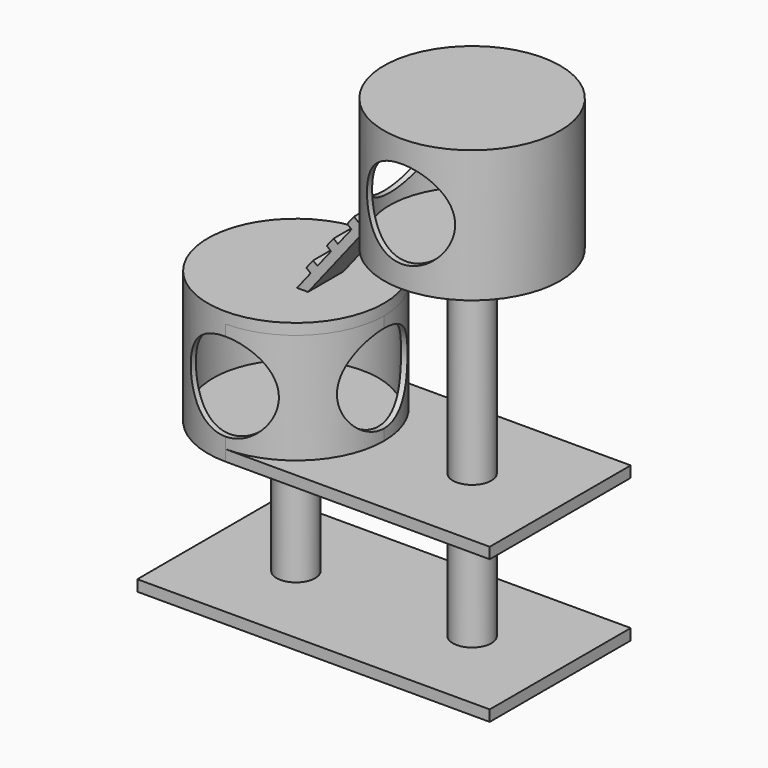
from build123d import *
from build123d import SkipClean  # not in build123d's __all__

# Parameters (mm, degrees)
F1_DEPTH  = 12.7
F2_R      = 44.45
F3_DEPTH  = 304.8
F4_W      = 812.8
F4_H      = 406.4
F5_DEPTH  = 25.4
F7_DEPTH  = 254
F8_R      = 190.5
F9_DEPTH  = 254
F10_R     = 101.6
F11_DEPTH = 205.74
F12_R     = 101.6
F13_DEPTH = 350.52
F14_R     = 203.2
F15_DEPTH = 25.4
F16_R     = 44.45
F17_DEPTH = 457.2
F18_R     = 203.2
F18_R_2   = 44.45
F19_DEPTH = 279.4
F20_R     = 190.5
F21_DEPTH = 254
F22_R     = 101.6
F23_DEPTH = 218.44
F24_R     = 101.6
F25_DEPTH = 393.7
F26_R     = 203.2
F27_DEPTH = 25.4
F29_DEPTH = 50.8
F30_W     = 101.6
F30_H     = 25.4
F31_DEPTH = 12.7


with BuildPart() as f1:
    # F0 (on Top) → F1 (new body, symmetric)
    with BuildSketch(Plane.XY):
        with BuildLine():
            Line((406.4, 203.2), (-203.2, 203.2))
            ThreePointArc((-203.2, 203.2), (-406.4, 0), (-203.2, -203.2))
            Line((-203.2, -203.2), (406.4, -203.2))
            Line((406.4, -203.2), (406.4, 203.2))
        make_face()
    extrude(amount=F1_DEPTH, both=True)

    # F2 (on face) → F3 (join)
    with BuildSketch(Plane(origin=(0, 0, -12.7), x_dir=(1, 0, 0), z_dir=(0, 0, -1))):
        with Locations((-203.2, 0)):
            Circle(F2_R)
        with Locations((203.2, 0)):
            Circle(F2_R)
    extrude(amount=F3_DEPTH)

    # F4 (on face) → F5 (join)
    with BuildSketch(Plane(origin=(0, 0, -317.5), x_dir=(1, 0, 0), z_dir=(0, 0, -1))):
        Rectangle(F4_W, F4_H)
    extrude(amount=F5_DEPTH)

    # F6 (on face) → F7 (join)
    with BuildSketch(Plane.XY.offset(12.7)):
        with BuildLine():
            ThreePointArc((-203.2, -203.2), (-59.515902, -143.684098), (0, 0))
            ThreePointArc((0, 0), (-59.515902, 143.684098), (-203.2, 203.2))
            ThreePointArc((-203.2, 203.2), (-406.4, 0), (-203.2, -203.2))
        make_face()
    extrude(amount=F7_DEPTH)

    # F8 (on face) → F9 (cut)
    with BuildSketch(Plane.XY.offset(266.7)):
        with Locations((-203.2, 0)):
            Circle(F8_R)
    extrude(amount=-F9_DEPTH, mode=Mode.SUBTRACT)

    # F10 (on Right) → F11 (cut)
    with BuildSketch(Plane.YZ):
        with Locations((0, 139.7)):
            Circle(F10_R)
    with SkipClean():  # cleaning this boolean's faces spoils the solid; the shape is the same uncleaned
        extrude(amount=-F11_DEPTH, mode=Mode.SUBTRACT)

    # F12 (on Front) → F13 (cut)
    with BuildSketch(Plane.XZ):
        with Locations((-203.2, 139.7)):
            Circle(F12_R)
    with SkipClean():  # cleaning this boolean's faces spoils the solid; the shape is the same uncleaned
        extrude(amount=F13_DEPTH, mode=Mode.SUBTRACT)

    # F14 (on face) → F15 (join)
    with BuildSketch(Plane.XY.offset(266.7)):
        with Locations((-203.2, 0)):
            Circle(F14_R)
    with SkipClean():  # cleaning this boolean's faces spoils the solid; the shape is the same uncleaned
        extrude(amount=F15_DEPTH)

    # F16 (on face) → F17 (join)
    with BuildSketch(Plane.XY.offset(12.7)):
        with Locations((203.2, 0)):
            Circle(F16_R)
    with SkipClean():  # cleaning this boolean's faces spoils the solid; the shape is the same uncleaned
        extrude(amount=F17_DEPTH)

    # F18 (on face) → F19 (join)
    with BuildSketch(Plane.XY.offset(469.9)):
        with Locations((203.2, 0)):
            Circle(F18_R)
        with Locations((203.2, 0)):
            Circle(F18_R_2, mode=Mode.SUBTRACT)
        with Locations((203.2, 0)):
            Circle(F18_R_2)
    with SkipClean():  # cleaning this boolean's faces spoils the solid; the shape is the same uncleaned
        extrude(amount=F19_DEPTH)

    # F20 (on face) → F21 (cut)
    with BuildSketch(Plane.XY.offset(749.3)):
        with Locations((203.2, 0)):
            Circle(F20_R)
    with SkipClean():  # cleaning this boolean's faces spoils the solid; the shape is the same uncleaned
        extrude(amount=-F21_DEPTH, mode=Mode.SUBTRACT)

    # F22 (on Right) → F23 (cut)
    with BuildSketch(Plane.YZ):
        with Locations((0, 622.3)):
            Circle(F22_R)
    with SkipClean():  # cleaning this boolean's faces spoils the solid; the shape is the same uncleaned
        extrude(amount=F23_DEPTH, mode=Mode.SUBTRACT)

    # F24 (on Front) → F25 (cut)
    with BuildSketch(Plane.XZ):
        with Locations((203.2, 622.3)):
            Circle(F24_R)
    with SkipClean():  # cleaning this boolean's faces spoils the solid; the shape is the same uncleaned
        extrude(amount=F25_DEPTH, mode=Mode.SUBTRACT)

    # F26 (on face) → F27 (join)
    with BuildSketch(Plane.XY.offset(749.3)):
        with Locations((203.2, 0)):
            Circle(F26_R)
    with SkipClean():  # cleaning this boolean's faces spoils the solid; the shape is the same uncleaned
        extrude(amount=F27_DEPTH)

    # F28 (on Front) → F29 (join, symmetric)
    with BuildSketch(Plane.XZ):
        Polygon((25.4, 495.3), (0, 495.3), (-159.976862, 292.1), (-134.576862, 292.1), align=None)
    extrude(amount=F29_DEPTH, both=True)

    # F30 (on face) → F31 (join)
    with BuildSketch(Plane(origin=(-240.732388, 0, 189.52565), x_dir=(0, -1, 0), z_dir=(-0.785717, 0, 0.618586))):
        with Locations((0, 194.048658)):
            Rectangle(F30_W, F30_H)
        with Locations((0, 270.248658)):
            Rectangle(F30_W, F30_H)
        with Locations((0, 346.448658)):
            Rectangle(F30_W, F30_H)
    extrude(amount=F31_DEPTH)


solid = f1.part
